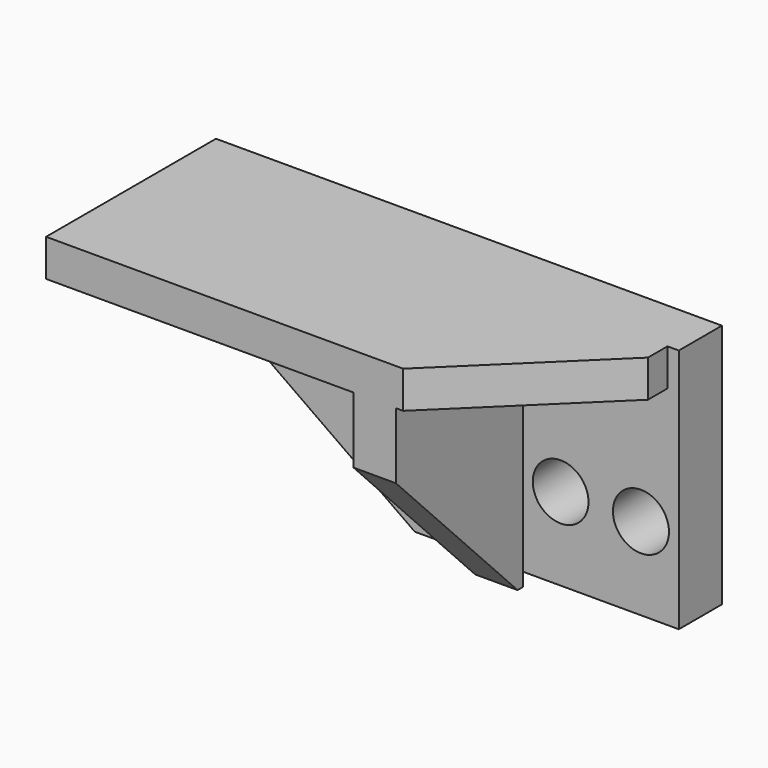
from build123d import *

# Parameters (mm, degrees)
F0_W      = 81.1027027667
F0_H      = 39.3372392282
F1_DEPTH  = 8.636
F3_DEPTH  = 25.4
F4_W      = 79.281533137
F4_H      = 5.9491507709
F5_DEPTH  = 25.4
F6_W      = 6.7990301177
F6_H      = 35.5734908953
F7_DEPTH  = 25.4
F9_DEPTH  = 25.4
F10_R     = 4.4646843998
F10_R_2   = 4.4902635422
F11_DEPTH = 25.4
F13_DEPTH = 25.4


with BuildPart() as f1:
    # F0 (on Front) → F1 (new body)
    with BuildSketch(Plane.XZ):
        with Locations((-8.7416078895, 6.434794981)):
            Rectangle(F0_W, F0_H)
    extrude(amount=F1_DEPTH)

    # F2 (on face) → F3 (cut)
    with BuildSketch(Plane.XZ.offset(8.636)):
        Polygon((-49.2929592729, -13.2338246331), (-10.5112984066, -13.2338246331), (-49.2929592729, 14.1543564849), align=None)
    extrude(amount=-F3_DEPTH, mode=Mode.SUBTRACT)

    # F4 (on face) → F5 (join)
    with BuildSketch(Plane.XZ.offset(8.636)):
        with Locations((-9.6521927044, 23.1288392097)):
            Rectangle(F4_W, F4_H)
    extrude(amount=F5_DEPTH)

    # F6 (on face) → F7 (join)
    with BuildSketch(Plane.XZ.offset(8.636)):
        with Locations((3.3995150588, 2.3675183766)):
            Rectangle(F6_W, F6_H)
    extrude(amount=F7_DEPTH)

    # F8 (on face) → F9 (cut)
    with BuildSketch(Plane.YZ.offset(6.7990301177)):
        Polygon((-34.036, -15.4192270711), (-9.674085426, -15.4192270711), (-34.036, 9.5568542875), align=None)
    extrude(amount=-F9_DEPTH, mode=Mode.SUBTRACT)

    # F10 (on face) → F11 (cut)
    with BuildSketch(Plane.XZ.offset(8.636)):
        with Locations((12.8695918247, 0)):
            Circle(F10_R)
        with Locations((25.7391780615, 0)):
            Circle(F10_R_2)
    extrude(amount=-F11_DEPTH, mode=Mode.SUBTRACT)

    # F12 (on face) → F13 (cut)
    with BuildSketch(Plane.XY.offset(26.1034145951)):
        Polygon((29.9885738641, -34.036), (29.9885738641, -12.5484813482), (7.9453402096, -34.036), align=None)
    extrude(amount=-F13_DEPTH, mode=Mode.SUBTRACT)


solid = f1.part
